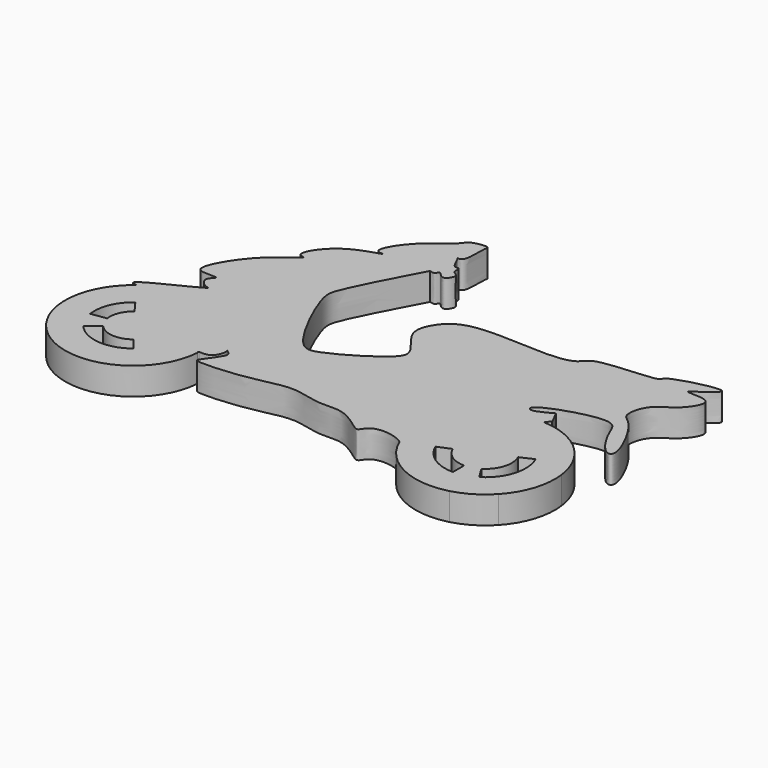
from build123d import *

# Parameters (mm, degrees)
F1_DEPTH = 3


with BuildPart() as f1:
    # F0 (on Top) → F1 (new body)
    with BuildSketch(Plane.XY):
        with BuildLine():
            add(Edge.make_bspline(
                [(13.7586910278, 24.360910058), (12.1445122128, 21.3203119824), (9.6921674336, 16.700876547), (9.4486919059, 14.5411167456), (13.3863253316, 6.2129092172), (15.964749388, 6.4060536096), (21.6030407466, 9.7954752322), (22.1872346086, 11.6399729397), (19.3782432715, 14.1900203006), (20.0421641979, 16.6354864615), (22.4642705762, 19.2775385675), (30.5715371437, 18.3052388587), (34.3640970115, 18.8334280632), (34.8247793369, 20.6519507648), (42.2249946892, 20.5637091519), (41.4982351867, 21.6514708245), (50.1586170845, 23.8241043222), (45.0747237582, 20.8130777783), (45.0910888553, 20.5099593857), (48.4704984618, 20.8523467626), (46.4222778313, 17.5058386781), (43.9994196037, 16.7325818251), (43.3692682581, 13.658778891), (45.0437982967, 13.2409039534), (47.8683361295, 7.8858885085), (46.6149125136, 7.0596071086), (44.3739891341, 10.3520567018), (44.0008884743, 13.101089161), (36.0250231226, 10.4973498656), (36.62178752, 9.2974405292), (37.870083582, 9.9518494869), (38.7683363129, 10.44651484)],
                knots=[0, 0, 0, 0, 0.0584173076, 0.0887506254, 0.1462882803, 0.1760248011, 0.2261989054, 0.2508727369, 0.2870727024, 0.3164581543, 0.3515889709, 0.4085193556, 0.4453651909, 0.4700753173, 0.5203838253, 0.5362502784, 0.5822959329, 0.6158667264, 0.6223329585, 0.6521687135, 0.6833865321, 0.7165574402, 0.746937641, 0.7721534539, 0.8192263814, 0.8346655334, 0.8723147778, 0.9023943696, 0.9550383992, 0.9681684105, 0.9976660926, 0.9976660926, 0.9976660926, 0.9976660926], degree=3))
            add(Edge.make_bspline(
                [(-4.2376262136, 6.5797739662), (-4.5536979814, 6.6193027908), (-5.9119655355, 6.789171553), (1.5738340505, 10.0989867355), (0.4139928611, 10.0171622462), (-0.7895353857, 11.1747535448), (0.8119222496, 12.1591675421), (-1.4678633347, 11.8720356841), (-2.3942079715, 12.7121940947), (0.4372262362, 17.5607629691), (4.1176243695, 19.5969839297), (3.4583987723, 19.5933486956), (2.6803787526, 19.947043912), (4.8146926793, 23.486016839), (9.6752756958, 24.4413321254), (7.1706619708, 24.1750575562), (9.5446688259, 28.0158614107), (12.4689842279, 29.5560076811), (12.9647325663, 30.8567663609), (15.0774259865, 31.0510514676), (14.7668880755, 30.4995455893), (15.029887143, 27.3768835667), (13.8836714306, 27.8124103572), (14.3415727307, 27.5925574823), (14.755658303, 26.0668814929), (15.6010221716, 26.4453171326), (15.2879753633, 25.3773271485), (16.410312065, 25.2511898587), (15.4508111543, 23.5126987041), (14.5046714047, 25.0236488051), (14.461627785, 24.1851683234), (14.0130867604, 24.2973083942), (13.7586910278, 24.360910058)],
                knots=[0, 0, 0, 0, 0.0220311323, 0.0946752453, 0.1102536014, 0.1438533687, 0.1705449832, 0.2058060245, 0.2319698118, 0.2995480168, 0.3532296207, 0.3669381734, 0.3870184903, 0.4429984813, 0.497083374, 0.5212159032, 0.5744033258, 0.6286372416, 0.6611743968, 0.6976275116, 0.7159732608, 0.7635510994, 0.7838936998, 0.7974040639, 0.8321047202, 0.8519760497, 0.8759166568, 0.9004649995, 0.9309726841, 0.9599148053, 0.9772651733, 1, 1, 1, 1], degree=3))
            ThreePointArc((-4.2376262136, 6.5797739662), (-3.4262249249, -6.0214012518), (7.6729063876, 0))
            add(Edge.make_bspline(
                [(7.6847799349, 0.2032470705), (7.6559692031, 0.1981725716), (7.5687413432, 0.1671127529), (7.6281408679, 0.0718176551), (7.6729063876, 0)],
                knots=[0.9841018197, 0.9841018197, 0.9841018197, 0.9841018197, 0.9880185859, 1, 1, 1, 1], degree=3))
            add(Edge.make_bspline(
                [(31.580850482, -2.0815322641), (30.5377129515, -1.3399234407), (27.9042836946, -1.1050092455), (27.4167243927, -2.815404507), (26.4269528276, -2.0448567791), (24.1512947622, -0.4261562344), (21.698776302, -0.9950019932), (18.1814471878, 0.3377397459), (14.2011175727, -1.0939501326), (8.3507483371, -1.4060057353), (8.5618748753, -0.8084421735), (9.9581985684, 0.9860523714), (9.9697282454, 1.552072044), (9.2794042921, 2.0392405198), (9.6137525273, 1.5949088623), (9.0530998241, 0.0544183172), (7.8748593036, 0.2367261763), (7.6847799349, 0.2032470705)],
                knots=[0.4415585238, 0.4415585238, 0.4415585238, 0.4415585238, 0.4935251535, 0.5233724666, 0.5493027128, 0.5950305399, 0.6382772431, 0.6893506722, 0.750253536, 0.8130183045, 0.8272158403, 0.8691745198, 0.8899311644, 0.9104113471, 0.9242534288, 0.9582608778, 0.9841018197, 0.9841018197, 0.9841018197, 0.9841018197], degree=3))
            add(Edge.make_bspline(
                [(40.6380668283, -6.5574813634), (38.6346604366, -6.9250075439), (33.5838139745, -6.3728783954), (32.7470610164, -2.910638683), (31.580850482, -2.0815322641)],
                knots=[0.3134003705, 0.3134003705, 0.3134003705, 0.3134003705, 0.38346069, 0.4415585238, 0.4415585238, 0.4415585238, 0.4415585238], degree=3))
            ThreePointArc((40.6380668283, -6.5574813634), (42.6153481703, -5.7186863551), (44.2822391626, -4.3641779604))
            add(Edge.make_bspline(
                [(46.2622994581, 1.8444166957), (46.2709457802, 1.6770408911), (46.3152349154, -0.5570978773), (45.4317626515, -2.8615756368), (44.3140043226, -4.3234938851), (44.2822391626, -4.3641779604)],
                knots=[0.182240108, 0.182240108, 0.182240108, 0.182240108, 0.1877184442, 0.2551516932, 0.2571081645, 0.2571081645, 0.2571081645, 0.2571081645], degree=3))
            ThreePointArc((46.2622994581, 1.8444166957), (45.3661366018, 4.5641141181), (43.5342676938, 6.7650498822))
            add(Edge.make_bspline(
                [(39.0784141577, 8.5008906299), (39.5818338302, 8.1963352444), (41.9455046445, 7.75411252), (43.5342676938, 6.7650498822)],
                knots=[0.0644672084, 0.0644672084, 0.0644672084, 0.0644672084, 0.119258273, 0.119258273, 0.119258273, 0.119258273], degree=3))
            add(Edge.make_bspline(
                [(38.9819815755, 8.6080878973), (38.9825163927, 8.5739384825), (39.0163097452, 8.5384621321), (39.0784141577, 8.5008906299)],
                knots=[0.0577079038, 0.0577079038, 0.0577079038, 0.0577079038, 0.0644672084, 0.0644672084, 0.0644672084, 0.0644672084], degree=3))
            add(Edge.make_bspline(
                [(39.2104805405, 8.8015334131), (39.0897206725, 8.7277423662), (38.9810103488, 8.670103147), (38.9819815755, 8.6080878973)],
                knots=[0.0454330241, 0.0454330241, 0.0454330241, 0.0454330241, 0.0577079038, 0.0577079038, 0.0577079038, 0.0577079038], degree=3))
            Line((39.2104805405, 8.8015334131), (39.4795835018, 9.0293539688))
            Line((39.4795835018, 9.0293539688), (38.7683363129, 10.44651484))
        make_face()
        with BuildLine():
            ThreePointArc((-4.0507202028, -0.0883874976), (-3.7652695752, 2.1931045174), (-2.3438051563, 4.0003473846))
            Line((-2.3438051563, 4.0003473846), (-1.3377127088, 2.6300269985))
            ThreePointArc((-1.3377127088, 2.6300269985), (-2.1966565095, 1.537777614), (-2.3688094383, 0.1589532815))
            ThreePointArc((-2.3688094203, 0.1589532842), (-2.1623539786, -0.5389853895), (-1.7701665596, -1.1521177325))
            Line((-1.7701665596, -1.1521177325), (0.1904377164, 0.5353146193))
            Line((0.1904377164, 0.5353146193), (0.1994143387, 0.536634716))
            Line((0.1994143387, 0.536634716), (1.8307144172, -1.4775270526))
            Line((1.8307144172, -1.4775270526), (2.9006636778, -2.7985904936))
            ThreePointArc((2.9006636778, -2.7985904936), (-0.1880123515, -3.7384920175), (-3.0586551198, -2.2610805702))
            ThreePointArc((-3.0586551198, -2.2610805702), (-3.7087740777, -1.2450908438), (-4.0507202028, -0.0883874976))
        make_face(mode=Mode.SUBTRACT)
        with BuildLine():
            ThreePointArc((38.6631296248, -3.6063057176), (36.1875731378, -2.8550180949), (34.5471130444, -0.8545922168))
            Line((34.5471130444, -0.8545922168), (35.9794210504, -0.2621443078))
            ThreePointArc((35.9794210504, -0.2621443078), (37.0490272419, -1.5664539423), (38.6631296248, -2.0563054761))
            Line((38.6631296248, -2.0563054761), (38.6631296248, -3.6063057176))
        make_face(mode=Mode.SUBTRACT)
        with BuildLine():
            ThreePointArc((40.2009012959, -1.6157735848), (39.462943675, -1.9440011407), (38.6631296248, -2.0563054761))
            Line((38.6631296248, -2.0563054761), (38.6631296248, 0.8479224702))
            Line((38.6631296248, 0.8479224702), (41.3072632416, 2.0492123522))
            Line((41.3072632416, 2.0492123522), (42.7184499047, 2.6903464648))
            ThreePointArc((42.7184499047, 2.6903464648), (42.927301441, -0.4393177834), (41.0216173367, -2.9306598647))
            Line((41.0216173367, -2.9306598647), (40.2009012959, -1.6157735848))
        make_face(mode=Mode.SUBTRACT)
        with BuildLine():
            Line((38.9819815755, 8.6080878973), (39.2104805405, 8.8015334131))
            add(Edge.make_bspline(
                [(39.2104805405, 8.8015334131), (39.0897206725, 8.7277423662), (38.9810103488, 8.670103147), (38.9819815755, 8.6080878973)],
                knots=[0.0454330241, 0.0454330241, 0.0454330241, 0.0454330241, 0.0577079038, 0.0577079038, 0.0577079038, 0.0577079038], degree=3))
        make_face()
        with BuildLine():
            Line((39.0784141577, 8.5008906299), (38.9819815755, 8.6080878973))
            add(Edge.make_bspline(
                [(38.9819815755, 8.6080878973), (38.9825163927, 8.5739384825), (39.0163097452, 8.5384621321), (39.0784141577, 8.5008906299)],
                knots=[0.0577079038, 0.0577079038, 0.0577079038, 0.0577079038, 0.0644672084, 0.0644672084, 0.0644672084, 0.0644672084], degree=3))
        make_face()
        with BuildLine():
            add(Edge.make_bspline(
                [(40.6380668283, -6.5574813634), (38.6346604366, -6.9250075439), (33.5838139745, -6.3728783954), (32.7470610164, -2.910638683), (31.580850482, -2.0815322641)],
                knots=[0.3134003705, 0.3134003705, 0.3134003705, 0.3134003705, 0.38346069, 0.4415585238, 0.4415585238, 0.4415585238, 0.4415585238], degree=3))
            ThreePointArc((31.580850482, -2.0815322641), (35.2675787849, -6.0230758117), (40.6380668283, -6.5574813634))
        make_face()
        with BuildLine():
            ThreePointArc((43.5342676938, 6.7650498822), (41.4451885309, 7.9893880859), (39.0784141577, 8.5008906299))
            add(Edge.make_bspline(
                [(39.0784141577, 8.5008906299), (39.5818338302, 8.1963352444), (41.9455046445, 7.75411252), (43.5342676938, 6.7650498822)],
                knots=[0.0644672084, 0.0644672084, 0.0644672084, 0.0644672084, 0.119258273, 0.119258273, 0.119258273, 0.119258273], degree=3))
        make_face()
        with BuildLine():
            add(Edge.make_bspline(
                [(46.2622994581, 1.8444166957), (46.2709457802, 1.6770408911), (46.3152349154, -0.5570978773), (45.4317626515, -2.8615756368), (44.3140043226, -4.3234938851), (44.2822391626, -4.3641779604)],
                knots=[0.182240108, 0.182240108, 0.182240108, 0.182240108, 0.1877184442, 0.2551516932, 0.2571081645, 0.2571081645, 0.2571081645, 0.2571081645], degree=3))
            ThreePointArc((44.2822391626, -4.3641779604), (45.9650053622, -1.4808097198), (46.2622994581, 1.8444166957))
        make_face()
        with BuildLine():
            Line((-2.3688094383, 0.1589532815), (-4.0507202028, -0.0883874976))
            ThreePointArc((-4.0507202028, -0.0883874976), (-3.7087740777, -1.2450908438), (-3.0586551198, -2.2610805702))
            Line((-3.0586551198, -2.2610805702), (-1.7701665596, -1.1521177325))
            ThreePointArc((-1.7701665596, -1.1521177325), (-2.1623539786, -0.5389853895), (-2.3688094203, 0.1589532842))
        make_face()
        with BuildLine():
            Line((0.1904377164, 0.5353146193), (-1.7701665596, -1.1521177325))
            ThreePointArc((-1.7701665596, -1.1521177325), (-0.0357411454, -2.0453252087), (1.8307144172, -1.4775270526))
            Line((1.8307144172, -1.4775270526), (0.1994143387, 0.536634716))
            Line((0.1994143387, 0.536634716), (0.1904377164, 0.5353146193))
        make_face()
        with BuildLine():
            Line((38.6631296248, 0.8479224702), (38.6631296248, -2.0563054761))
            ThreePointArc((38.6631296248, -2.0563054761), (39.462943675, -1.9440011407), (40.2009012959, -1.6157735848))
            Line((40.2009012959, -1.6157735848), (38.6631296248, 0.8479224702))
        make_face()
        with BuildLine():
            Line((41.3072632416, 2.0492123522), (38.6631296248, 0.8479224702))
            Line((38.6631296248, 0.8479224702), (40.2009012959, -1.6157735848))
            ThreePointArc((40.2009012959, -1.6157735848), (41.4434377801, 0.0086212578), (41.3072632416, 2.0492123522))
        make_face()
    extrude(amount=F1_DEPTH)


solid = f1.part
